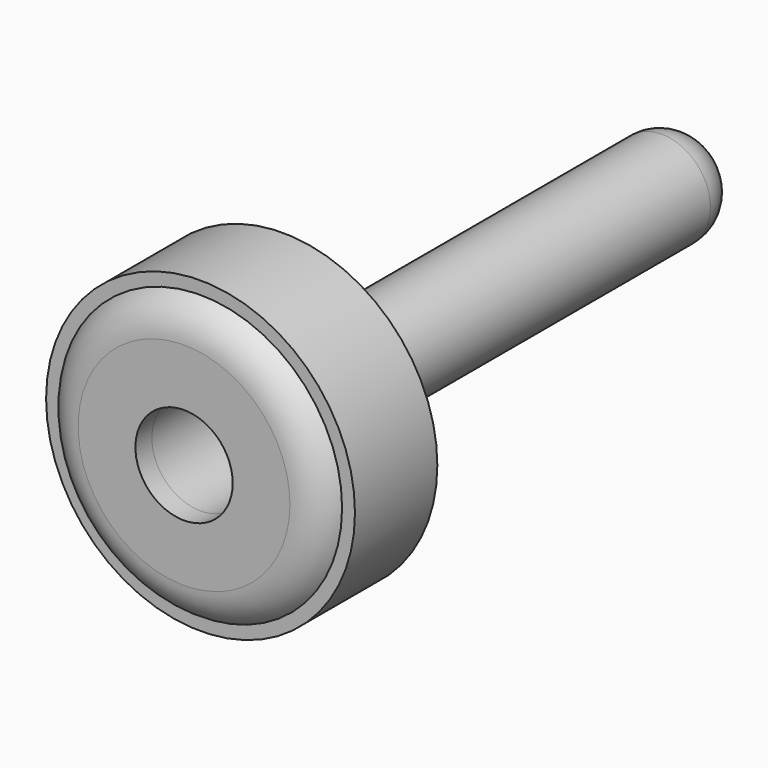
from build123d import *

# Parameters (mm, degrees)
F0_R     = 6
F1_DEPTH = 63.5
F2_R     = 19.05
F2_R_2   = 6
F3_DEPTH = 12.7
F4_R     = 17.4625
F4_R_2   = 6
F5_DEPTH = 2.54
F6_R     = 5.08


# Not quite as in the source:
# - a fillet or chamfer that OpenCascade refuses, or shapes differently, is made with other operations: its cross-section is extruded or revolved along the edge and cut away or added


with BuildPart() as f1:
    # F0 (on Front) → F1 (new body)
    with BuildSketch(Plane.XZ):
        Circle(F0_R)
    extrude(amount=F1_DEPTH)

    # F6
    f6_edges = [f1.edges().sort_by_distance(p)[0] for p in [
        (-6, 0, 0),
    ]]
    fillet(f6_edges, radius=F6_R)


with BuildPart() as f3:
    # F2 (on face) → F3 (new body)
    with BuildSketch(Plane.XZ.offset(63.5)):
        Circle(F2_R)
        Circle(F2_R_2, mode=Mode.SUBTRACT)
    extrude(amount=F3_DEPTH)


with BuildPart() as f5:
    # F4 (on face) → F5 (new body)
    with BuildSketch(Plane.XZ.offset(76.2)):
        Circle(F4_R)
        Circle(F4_R_2, mode=Mode.SUBTRACT)
    extrude(amount=F5_DEPTH)

    # F7: fillet of radius 5.08 on 1 edges, made by hand

    # F7_s1 → F7_t2 (revolve, cut)
    with BuildSketch(Plane.XY):
        with BuildLine():
            ThreePointArc((17.4625, -76.2), (15.6030909488, -78.0594090512), (13.0630909488, -78.74))
            Line((13.0630909488, -78.74), (17.4625, -78.74))
            Line((17.4625, -78.74), (17.4625, -76.2))
        make_face()
    revolve(axis=Axis((0, -78.74, 0), (0, -1, 0)), mode=Mode.SUBTRACT)


solid = Compound([f1.part, f3.part, f5.part])
